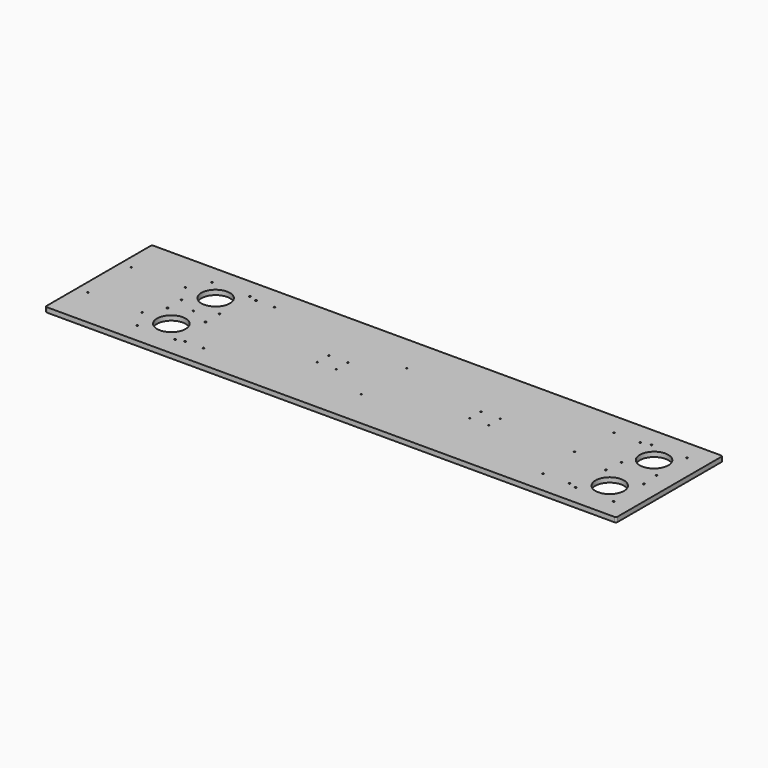
from build123d import *

# Parameters (mm, degrees)
F0_R     = 1.7272
F1_DEPTH = 12.7
F2_R     = 1.7272
F2_R_2   = 38.1
F2_R_3   = 2.15265
F3_DEPTH = 12.7
F4_R     = 1.7272
F4_R_2   = 2.15265
F5_DEPTH = 12.7
F6_R     = 3.96875
F7_DEPTH = 6.35
F8_R     = 3.96875


# Not quite as in the source:
# - a feature names something its author has since deleted; it is built from what else it names


with BuildPart() as f1:
    # F0 (on Top) → F1 (new body)
    with BuildSketch(Plane.XY):
        Polygon((0, -177.8), (0, 0), (0, 177.8), (-1524, 177.8), (-1524, -177.8), align=None)
        with Locations((-1494.63125, -72.23125)):
            Circle(F0_R, mode=Mode.SUBTRACT)
        with Locations((-1350.16875, -72.23125)):
            Circle(F0_R, mode=Mode.SUBTRACT)
        with Locations((-1494.63125, 72.23125)):
            Circle(F0_R, mode=Mode.SUBTRACT)
        with Locations((-1350.16875, 72.23125)):
            Circle(F0_R, mode=Mode.SUBTRACT)
    extrude(amount=F1_DEPTH)

    # F2 (on face) → F3 (cut, through all)
    with BuildSketch(Plane.XY.offset(12.7)):
        with Locations((-1270.635, 0)):
            Circle(F2_R)
        with Locations((-762, -75.565)):
            Circle(F2_R)
        with Locations((-762, 75.565)):
            Circle(F2_R)
        with Locations((-253.365, 0)):
            Circle(F2_R)
        with Locations((-100.1617631794, 73.9775)):
            Circle(F2_R_2)
        with Locations((-100.1617631794, -73.9775)):
            Circle(F2_R_2)
        with Locations((-1270.635, 73.9775)):
            Circle(F2_R_2)
        with Locations((-1270.635, -73.9775)):
            Circle(F2_R_2)
        with Locations((-150.7879570619, -124.6036938825)):
            Circle(F2_R_3)
        with Locations((-49.5355692968, -124.6036938825)):
            Circle(F2_R_3)
        with Locations((-49.5355692968, -23.3513061175)):
            Circle(F2_R_3)
        with Locations((-150.7879570619, -23.3513061175)):
            Circle(F2_R_3)
        with Locations((-147.1272202412, 23.3513061175)):
            Circle(F2_R_3)
        with Locations((-147.1272202412, 124.6036938825)):
            Circle(F2_R_3)
        with Locations((-53.1963061175, 124.6036938825)):
            Circle(F2_R_3)
        with Locations((-53.1963061175, 23.3513061175)):
            Circle(F2_R_3)
        with Locations((-1321.2611938825, -124.6036938825)):
            Circle(F2_R_3)
        with Locations((-1220.0088061175, -124.6036938825)):
            Circle(F2_R_3)
        with Locations((-1220.0088061175, -23.3513061175)):
            Circle(F2_R_3)
        with Locations((-1321.2611938825, -23.3513061175)):
            Circle(F2_R_3)
        with Locations((-1321.2611938825, 23.3513061175)):
            Circle(F2_R_3)
        with Locations((-1220.0088061175, 23.3513061175)):
            Circle(F2_R_3)
        with Locations((-1220.0088061175, 124.6036938825)):
            Circle(F2_R_3)
        with Locations((-1321.2611938825, 124.6036938825)):
            Circle(F2_R_3)
    extrude(amount=-F3_DEPTH, mode=Mode.SUBTRACT)

    # F4 (on face) → F5 (cut, through all)
    with BuildSketch(Plane.XY.offset(12.7)):
        with Locations((-467.2984367897, -19.05)):
            Circle(F4_R)
        with Locations((-518.0984367897, -19.05)):
            Circle(F4_R)
        with Locations((-518.0984367897, 19.05)):
            Circle(F4_R)
        with Locations((-467.2984367897, 19.05)):
            Circle(F4_R)
        with Locations((-873.6984367897, 19.05)):
            Circle(F4_R)
        with Locations((-873.6984367897, -19.05)):
            Circle(F4_R)
        with Locations((-924.4984367897, -19.05)):
            Circle(F4_R)
        with Locations((-924.4984367897, 19.05)):
            Circle(F4_R)
        with Locations((-172.5517631794, 118.3676195)):
            Circle(F4_R_2)
        with Locations((-242.2869805794, 118.3676195)):
            Circle(F4_R_2)
        with Locations((-242.2869805794, -118.3676195)):
            Circle(F4_R_2)
        with Locations((-172.5517631794, -118.3676195)):
            Circle(F4_R_2)
        with Locations((-1198.245, -118.3676195)):
            Circle(F4_R_2)
        with Locations((-1149.509893, -118.3676195)):
            Circle(F4_R_2)
        with Locations((-1198.245, 118.3676195)):
            Circle(F4_R_2)
        with Locations((-1149.509893, 118.3676195)):
            Circle(F4_R_2)
    extrude(amount=-F5_DEPTH, mode=Mode.SUBTRACT)

    # F6 (on face) → F7 (cut)
    with BuildSketch(Plane(origin=(0, 0, 0), x_dir=(1, 0, 0), z_dir=(0, 0, -1))):
        with Locations((-924.4984367897, -19.05)):
            Circle(F6_R)
        with Locations((-873.6984367897, -19.05)):
            Circle(F6_R)
        with Locations((-873.6984367897, 19.05)):
            Circle(F6_R)
        with Locations((-924.4984367897, 19.05)):
            Circle(F6_R)
        with Locations((-467.2984367897, -19.05)):
            Circle(F6_R)
        with Locations((-467.2984367897, 19.05)):
            Circle(F6_R)
        with Locations((-518.0984367897, 19.05)):
            Circle(F6_R)
        with Locations((-518.0984367897, -19.05)):
            Circle(F6_R)
    extrude(amount=-F7_DEPTH, mode=Mode.SUBTRACT)

    # F8
    f8_edges = [f1.edges().sort_by_distance(p)[0] for p in [
        (-1524, 177.8, 6.35),
        (-1524, -177.8, 6.35),
        (0, -177.8, 6.35),
        (0, 177.8, 6.35),
    ]]
    fillet(f8_edges, radius=F8_R)


solid = f1.part
